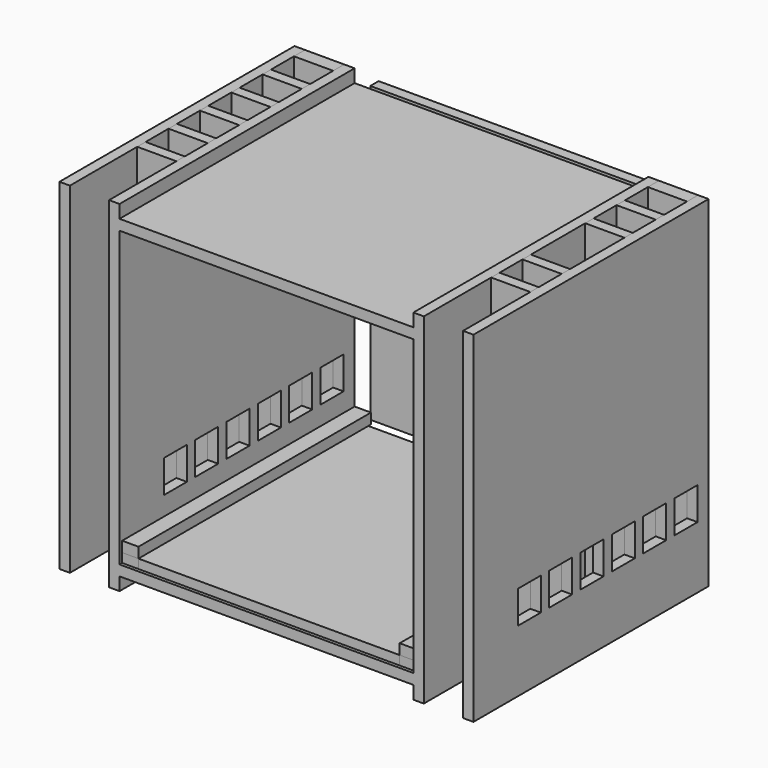
from build123d import *

# Parameters (mm, degrees)
F1_W          = 450
F1_H          = 16
F3_DEPTH      = 450
F1_W_2        = 16
F1_H_2        = 522
F4_W          = 44
F4_H          = 50
F5_DEPTH      = 1209
F5_DEPTH_BACK = 175
F6_W          = 60
F6_H          = 21.131195128
F7_DEPTH      = 572
F6_H_2        = 16
F7_FACE_W     = 60
F7_FACE_H     = 21.131195128
F7_FACE_H_2   = 16
F8_DEPTH      = 50
F9_START      = -30
F1_H_3        = 450
F9_DEPTH      = 16
F11_START     = 86
F11_DEPTH     = 14
F12_START     = 70
F10_W         = 25
F10_H         = 20
F12_DEPTH     = 30
F13_W         = 25
F13_H         = 16
F14_DEPTH     = 445


with BuildPart() as f3:
    # F1 (on Front) → F3 (new body, through all)
    with BuildSketch(Plane.XZ):
        with Locations((291, 78)):
            Rectangle(F1_W, F1_H)
        Polygon((516, 86), (516, 70), (516, 50), (532, 50), (532, 572), (516, 572), (516, 552), (516, 536), align=None)
        with Locations((291, 544)):
            Rectangle(F1_W, F1_H)
        Polygon((50, 572), (50, 50), (66, 50), (66, 70), (66, 86), (66, 536), (66, 552), (66, 572), align=None)
    extrude(amount=F3_DEPTH)


with BuildPart() as f3b:
    # F1 (on Front) → F3, piece 2 (new body, through all)
    with BuildSketch(Plane.XZ):
        with Locations((600, 311)):
            Rectangle(F1_W_2, F1_H_2)
    extrude(amount=F3_DEPTH)


with BuildPart() as f3c:
    # F1 (on Front) → F3, piece 3 (new body, through all)
    with BuildSketch(Plane.XZ):
        with Locations((-18, 311)):
            Rectangle(F1_W_2, F1_H_2)
    extrude(amount=F3_DEPTH)


with BuildPart() as f5_tool:
    # F4 (on Right) → F5 (new body, two sides)
    with BuildSketch(Plane.YZ) as f5_sk:
        with Locations((-43.131195128, 170)):
            Rectangle(F4_W, F4_H)
        with Locations((-103.131195128, 170)):
            Rectangle(F4_W, F4_H)
        with Locations((-163.131195128, 170)):
            Rectangle(F4_W, F4_H)
        with Locations((-223.131195128, 170)):
            Rectangle(F4_W, F4_H)
        with Locations((-283.131195128, 170)):
            Rectangle(F4_W, F4_H)
        with Locations((-343.131195128, 170)):
            Rectangle(F4_W, F4_H)
    extrude(amount=F5_DEPTH)
    extrude(f5_sk.sketch, amount=-F5_DEPTH_BACK)


with BuildPart() as f3_1:
    add(f3.part)

    # F5: cut by f5_tool
    add(f5_tool.part, mode=Mode.SUBTRACT)

    # F10 (on Top) → F12 (join)
    with BuildSketch(Plane.XY.offset(F12_START)):
        with Locations((78.5, -435)):
            Rectangle(F10_W, F10_H)
        with Locations((503.5, -435)):
            Rectangle(F10_W, F10_H)
    extrude(amount=F12_DEPTH)


with BuildPart() as f3b_1:
    add(f3b.part)

    # F5: cut by f5_tool
    add(f5_tool.part, mode=Mode.SUBTRACT)


with BuildPart() as f3c_1:
    add(f3c.part)

    # F5: cut by f5_tool
    add(f5_tool.part, mode=Mode.SUBTRACT)


with BuildPart() as f7:
    # F6 (on Top) → F7 (new body, through all)
    with BuildSketch(Plane.XY):
        with Locations((20, -10.565597564)):
            Rectangle(F6_W, F6_H)
    extrude(amount=F7_DEPTH)


with BuildPart() as f7b:
    # F6 (on Top) → F7, piece 2 (new body, through all)
    with BuildSketch(Plane.XY):
        with Locations((20, -73.131195128)):
            Rectangle(F6_W, F6_H_2)
    extrude(amount=F7_DEPTH)


with BuildPart() as f7c:
    # F6 (on Top) → F7, piece 3 (new body, through all)
    with BuildSketch(Plane.XY):
        with Locations((20, -133.131195128)):
            Rectangle(F6_W, F6_H_2)
    extrude(amount=F7_DEPTH)


with BuildPart() as f7d:
    # F6 (on Top) → F7, piece 4 (new body, through all)
    with BuildSketch(Plane.XY):
        with Locations((20, -193.131195128)):
            Rectangle(F6_W, F6_H_2)
    extrude(amount=F7_DEPTH)


with BuildPart() as f7e:
    # F6 (on Top) → F7, piece 5 (new body, through all)
    with BuildSketch(Plane.XY):
        with Locations((20, -253.131195128)):
            Rectangle(F6_W, F6_H_2)
    extrude(amount=F7_DEPTH)


with BuildPart() as f7f:
    # F6 (on Top) → F7, piece 6 (new body, through all)
    with BuildSketch(Plane.XY):
        with Locations((20, -313.131195128)):
            Rectangle(F6_W, F6_H_2)
    extrude(amount=F7_DEPTH)


with BuildPart() as f7g:
    # F6 (on Top) → F7, piece 7 (new body, through all)
    with BuildSketch(Plane.XY):
        with Locations((562, -313.131195128)):
            Rectangle(F6_W, F6_H_2)
    extrude(amount=F7_DEPTH)


with BuildPart() as f7h:
    # F6 (on Top) → F7, piece 8 (new body, through all)
    with BuildSketch(Plane.XY):
        with Locations((562, -253.131195128)):
            Rectangle(F6_W, F6_H_2)
    extrude(amount=F7_DEPTH)


with BuildPart() as f7i:
    # F6 (on Top) → F7, piece 9 (new body, through all)
    with BuildSketch(Plane.XY):
        with Locations((562, -133.131195128)):
            Rectangle(F6_W, F6_H_2)
    extrude(amount=F7_DEPTH)


with BuildPart() as f7j:
    # F6 (on Top) → F7, piece 10 (new body, through all)
    with BuildSketch(Plane.XY):
        with Locations((562, -73.131195128)):
            Rectangle(F6_W, F6_H_2)
    extrude(amount=F7_DEPTH)


with BuildPart() as f7k:
    # F6 (on Top) → F7, piece 11 (new body, through all)
    with BuildSketch(Plane.XY):
        with Locations((562, -10.565597564)):
            Rectangle(F6_W, F6_H)
    extrude(amount=F7_DEPTH)


with BuildPart() as f8_tool:
    # F7_face (on face) → F8 (new body, through all)
    with BuildSketch(Plane(origin=(20, -10.565597564, 0), x_dir=(1, 0, 0), z_dir=(0, 0, -1))):
        Rectangle(F7_FACE_W, F7_FACE_H)
        with Locations((0, 62.565597564)):
            Rectangle(F7_FACE_W, F7_FACE_H_2)
        with Locations((0, 122.565597564)):
            Rectangle(F7_FACE_W, F7_FACE_H_2)
        with Locations((0, 182.565597564)):
            Rectangle(F7_FACE_W, F7_FACE_H_2)
        with Locations((0, 242.565597564)):
            Rectangle(F7_FACE_W, F7_FACE_H_2)
        with Locations((0, 302.565597564)):
            Rectangle(F7_FACE_W, F7_FACE_H_2)
        with Locations((542, 0)):
            Rectangle(F7_FACE_W, F7_FACE_H)
        with Locations((542, 62.565597564)):
            Rectangle(F7_FACE_W, F7_FACE_H_2)
        with Locations((542, 122.565597564)):
            Rectangle(F7_FACE_W, F7_FACE_H_2)
        with Locations((542, 242.565597564)):
            Rectangle(F7_FACE_W, F7_FACE_H_2)
        with Locations((542, 302.565597564)):
            Rectangle(F7_FACE_W, F7_FACE_H_2)
    extrude(amount=-F8_DEPTH)


with BuildPart() as f7_1:
    add(f7.part)

    # F8: cut by f8_tool
    add(f8_tool.part, mode=Mode.SUBTRACT)


with BuildPart() as f7b_1:
    add(f7b.part)

    # F8: cut by f8_tool
    add(f8_tool.part, mode=Mode.SUBTRACT)


with BuildPart() as f7c_1:
    add(f7c.part)

    # F8: cut by f8_tool
    add(f8_tool.part, mode=Mode.SUBTRACT)


with BuildPart() as f7d_1:
    add(f7d.part)

    # F8: cut by f8_tool
    add(f8_tool.part, mode=Mode.SUBTRACT)


with BuildPart() as f7e_1:
    add(f7e.part)

    # F8: cut by f8_tool
    add(f8_tool.part, mode=Mode.SUBTRACT)


with BuildPart() as f7f_1:
    add(f7f.part)

    # F8: cut by f8_tool
    add(f8_tool.part, mode=Mode.SUBTRACT)


with BuildPart() as f7g_1:
    add(f7g.part)

    # F8: cut by f8_tool
    add(f8_tool.part, mode=Mode.SUBTRACT)


with BuildPart() as f7h_1:
    add(f7h.part)

    # F8: cut by f8_tool
    add(f8_tool.part, mode=Mode.SUBTRACT)


with BuildPart() as f7i_1:
    add(f7i.part)

    # F8: cut by f8_tool
    add(f8_tool.part, mode=Mode.SUBTRACT)


with BuildPart() as f7j_1:
    add(f7j.part)

    # F8: cut by f8_tool
    add(f8_tool.part, mode=Mode.SUBTRACT)


with BuildPart() as f7k_1:
    add(f7k.part)

    # F8: cut by f8_tool
    add(f8_tool.part, mode=Mode.SUBTRACT)


with BuildPart() as f9:
    # F1 (on Front) → F9 (new body)
    with BuildSketch(Plane.XZ.offset(F9_START)):
        with Locations((291, 311)):
            Rectangle(F1_W, F1_H_3)
    extrude(amount=-F9_DEPTH)


with BuildPart() as f11:
    # F10 (on Top) → F11 (new body)
    with BuildSketch(Plane.XY.offset(F11_START)):
        Polygon((491, -25), (91, -25), (91, -425), (91, -445), (491, -445), (491, -425), align=None)
        Polygon((66, -5), (66, -25), (91, -25), (491, -25), (516, -25), (516, -5), align=None)
    extrude(amount=F11_DEPTH)


with BuildPart() as f14:
    # F13 (on face) → F14 (new body, through all)
    with BuildSketch(Plane.XZ.offset(445)):
        with Locations((78.5, 108)):
            Rectangle(F13_W, F13_H)
    extrude(amount=-F14_DEPTH)


with BuildPart() as f14b:
    # F13 (on face) → F14, piece 2 (new body, through all)
    with BuildSketch(Plane.XZ.offset(445)):
        with Locations((503.5, 108)):
            Rectangle(F13_W, F13_H)
    extrude(amount=-F14_DEPTH)


solid = Compound([f3_1.part, f3b_1.part, f3c_1.part, f7_1.part, f7b_1.part, f7c_1.part, f7d_1.part, f7e_1.part, f7f_1.part, f7g_1.part, f7h_1.part, f7i_1.part, f7j_1.part, f7k_1.part, f9.part, f11.part, f14.part, f14b.part])
